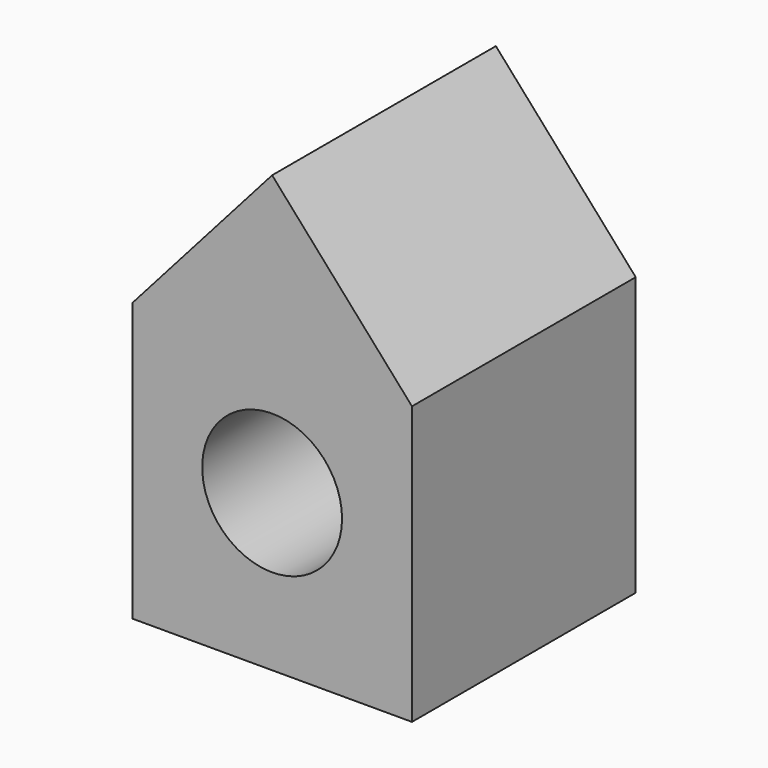
from build123d import *

# Parameters (mm, degrees)
F1_W     = 25.4
F1_H     = 25.2323417494
F2_DEPTH = 25.4
F3_R     = 6.35
F4_DEPTH = 16.9333333333


# Not quite as in the source:
# - the program builds the solid bodies; features that only make, move or delete a surface that nothing else refers to are left out


with BuildPart() as f2:
    # F1 (on Front) → F2 (new body)
    with BuildSketch(Plane.XZ):
        Polygon((12.7, 39.5754580502), (0, 25.2323417494), (25.4, 25.2323417494), align=None)
        with Locations((12.7, 12.6161708747)):
            Rectangle(F1_W, F1_H)
    extrude(amount=-F2_DEPTH)

    # F3 (on face) → F4 (cut)
    with BuildSketch(Plane.XZ):
        with Locations((12.7, 14.1754580502)):
            Circle(F3_R)
    extrude(amount=-F4_DEPTH, mode=Mode.SUBTRACT)


solid = f2.part
